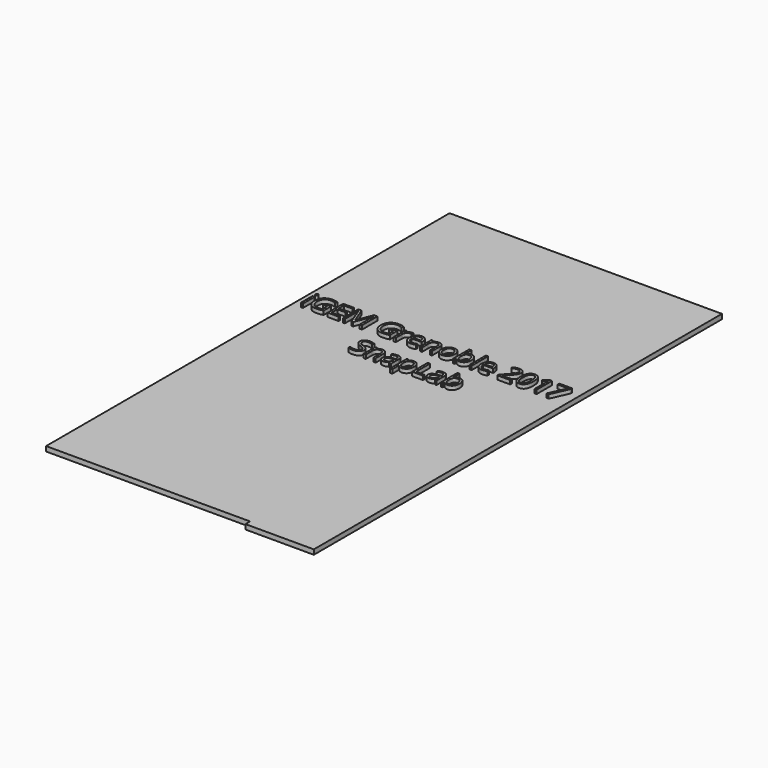
from build123d import *

# Parameters (mm, degrees)
F1_DEPTH     = 2.5
F2_TEXT_SIZE = 14.0588388441
F3_DEPTH     = 2


# Not quite as in the source:
# - Text() gives the source's letters only with a copy of the font that has no kerning and outlines rounded to 1/6400 em; it was checked with that copy


with BuildPart() as f1:
    # F0 (on Top) → F1 (new body)
    with BuildSketch(Plane.XY):
        Polygon((0, 262), (0, 0), (106, 0), (106, -3), (141.5, -3), (141.5, 262), align=None)
    extrude(amount=F1_DEPTH)

    # F2 (on face) → F3 (join)
    with BuildSketch(Plane.XY.offset(2.5)):
        with Locations((3.25, 159.8776360323)):
            Text('iGEM Grenoble 2017', F2_TEXT_SIZE, font='Open Sans', text_align=(TextAlign.LEFT, TextAlign.BOTTOM))
        with Locations((43.4341154647, 140.7576152044)):
            Text('SnapLab', F2_TEXT_SIZE, font='Open Sans', text_align=(TextAlign.LEFT, TextAlign.BOTTOM))
    extrude(amount=F3_DEPTH)


solid = f1.part
